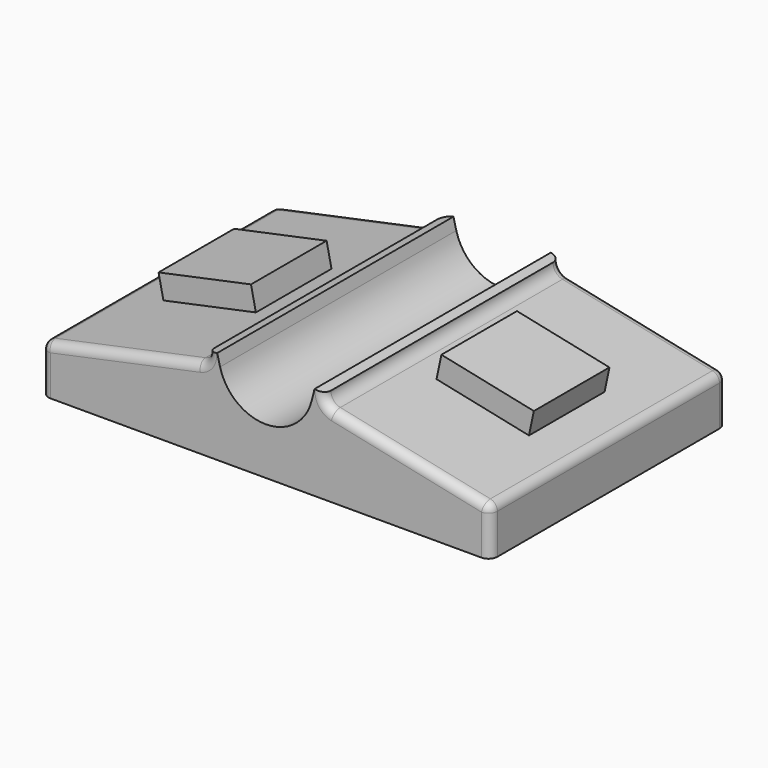
from build123d import *

# Parameters (mm, degrees)
F1_DEPTH    = 6.35
F4_T1_DEPTH = 6.35
F2_W        = 2.032
F2_H        = 2.032
F5_DEPTH    = 0.508
F7_R        = 0.1905
F12_DEPTH   = 0.254


# Not quite as in the source:
# - a fillet or chamfer that OpenCascade refuses, or shapes differently, is made with other operations: its cross-section is extruded or revolved along the edge and cut away or added


with BuildPart() as f1:
    # F0 (on Front) → F1 (new body)
    with BuildSketch(Plane.XZ):
        with BuildLine():
            Line((0, 0.7623671392), (0, 0))
            Line((0, 0), (9.652, 0))
            Line((9.652, 0), (9.652, 0.7623671392))
            Line((9.652, 0.7623671392), (6.0225553446, 1.5280881198))
            Line((6.0225553446, 1.5280881198), (6.0735776823, 1.729142969))
            Line((6.0735776823, 1.729142969), (5.8725685775, 1.7715508037))
            Line((5.8725685775, 1.7715508037), (5.8107842668, 1.5280881198))
            ThreePointArc((5.8107842668, 1.5280881198), (4.826, 0.762), (3.8412157332, 1.5280881198))
            Line((3.8412157332, 1.5280881198), (3.7794314225, 1.7715508037))
            Line((3.7794314225, 1.7715508037), (3.5784223177, 1.729142969))
            Line((3.5784223177, 1.729142969), (3.6294446554, 1.5280881198))
            Line((3.6294446554, 1.5280881198), (0, 0.7623671392))
        make_face()
    extrude(amount=-F1_DEPTH)

    # F4: fillet of radius 0.254 on 2 edges, made by hand

    # F4_s2 → F4_t1 (join)
    with BuildSketch(Plane.XZ.offset(-6.35)):
        with BuildLine():
            ThreePointArc((6.2750780534, 1.4748122183), (6.1284229129, 1.5656081597), (6.0735776823, 1.729142969))
            Line((6.0735776823, 1.729142969), (6.0225553446, 1.5280881198))
            Line((6.0225553446, 1.5280881198), (6.2750780534, 1.4748122183))
        make_face()
        with BuildLine():
            ThreePointArc((3.5784223177, 1.729142969), (3.5235770871, 1.5656081597), (3.3769219466, 1.4748122183))
            Line((3.3769219466, 1.4748122183), (3.6294446554, 1.5280881198))
            Line((3.6294446554, 1.5280881198), (3.5784223177, 1.729142969))
        make_face()
    extrude(amount=F4_T1_DEPTH)

    # F2 (on face) → F5 (join)
    with BuildSketch(Plane(origin=(0.5652924546, 0, 2.6794324958), x_dir=(0.9784612522, 0, -0.2064305646), z_dir=(0.2064305646, 0, 0.9784612522))):
        with Locations((7.3553929503, 3.175)):
            Rectangle(F2_W, F2_H)
    f5 = extrude(amount=F5_DEPTH)

    # F6: F5 across plane
    add(f5.mirror(Plane.YZ.offset(4.826)))

    # F7
    f7_edges = [f1.edges().sort_by_distance(p)[0] for p in [
        (9.652, 3.175, 0.762367),
        (0, 3.175, 0.762367),
        (7.963539, 6.35, 1.11859),
        (7.963539, 0, 1.11859),
        (1.688461, 0, 1.11859),
        (1.688461, 6.35, 1.11859),
        (9.652, 0, 0.381184),
        (9.652, 6.35, 0.381184),
        (0, 0, 0.381184),
        (0, 6.35, 0.381184),
        (3.523577, 6.35, 1.565608),
        (3.523577, 0, 1.565608),
        (6.128423, 0, 1.565608),
        (6.128423, 6.35, 1.565608),
    ]]
    fillet(f7_edges, radius=F7_R)


with BuildPart() as f8_1:
    # F8: copy of F1
    add(f1.part)


with BuildPart() as f9_1:
    # F9: copy of F8_1
    add(f8_1.part)


with BuildPart() as f1_1:
    add(f1.part)

    # F12 (add): a face of the model
    f12_faces = [f1_1.faces().sort_by_distance(p)[0] for p in [
        (4.826, 3.175, 0),
    ]]
    extrude(f12_faces, amount=F12_DEPTH)


solid = f1_1.part
